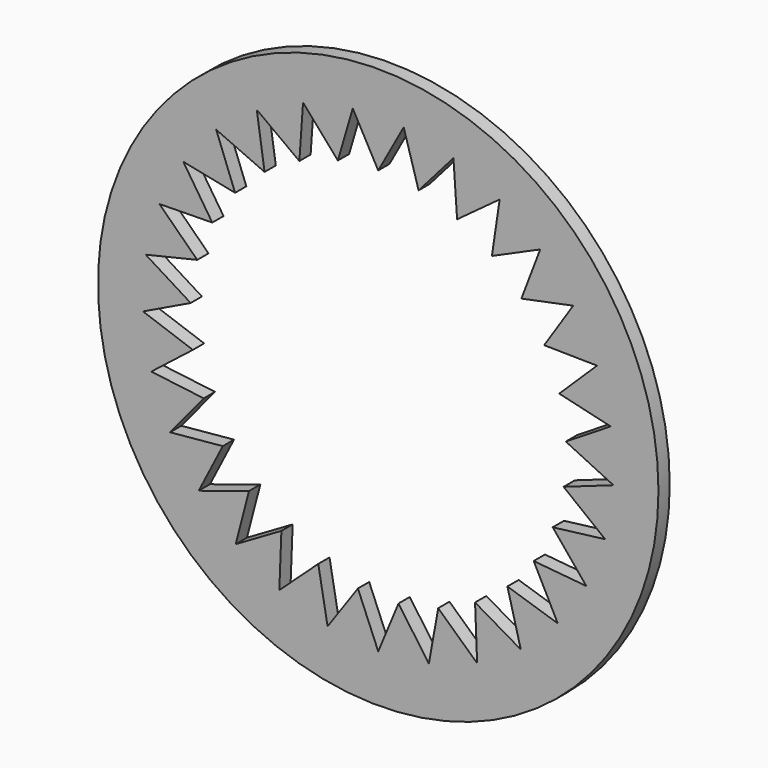
from build123d import *

# Parameters (mm, degrees)
F0_R     = 59.69
F1_DEPTH = 3


# Not quite as in the source:
# - a feature names something its author has since deleted; it is built from what else it names


with BuildPart() as f1:
    # F0 (on Front) → F1 (new body)
    with BuildSketch(Plane.XZ):
        Circle(F0_R)
        Polygon((-5.4242289373, 50.5095806797), (0, 40.6400127475), (5.4242289373, 50.5095806797), (8.5999770533, 39.7047088787), (16.0190558954, 48.1774829148), (16.7978287377, 36.9425310416), (25.8648496037, 43.6223336845), (24.2102326198, 32.482635602), (34.5012316912, 37.0571267042), (30.4905929324, 26.5335623138), (41.5243745303, 28.7888437555), (35.3452470073, 19.3734832321), (46.6058837673, 19.2041005596), (38.5471966155, 11.3371956968), (49.5081536781, 8.7510690557), (39.9467221522, 2.8004675814), (50.0954773473, -2.0814786208), (39.4783833586, -5.8375331953), (48.3403921728, -12.7870245801), (37.1640792362, -14.1729033174), (44.3249639868, -22.8649893915), (33.1120240736, -21.8158901421), (38.2369497485, -31.8441386213), (27.5116874668, -28.4091161002), (30.3610182372, -39.304617231), (20.624934931, -33.6442892735), (21.065439257, -44.8975815327), (12.7737833608, -37.2766187831), (10.7848637497, -48.3615107316), (4.3253438778, -39.136260938), (0, -49.5344353485), (-4.3253438778, -39.136260938), (-10.7848637497, -48.3615107316), (-12.7737833608, -37.2766187831), (-21.065439257, -44.8975815327), (-20.624934931, -33.6442892735), (-30.3610182372, -39.304617231), (-27.5116874668, -28.4091161002), (-38.2369497485, -31.8441386213), (-33.1120240736, -21.8158901421), (-44.3249639868, -22.8649893915), (-37.1640792362, -14.1729033174), (-48.3403921728, -12.7870245801), (-39.4783833586, -5.8375331953), (-50.0954773473, -2.0814786208), (-39.9467221522, 2.8004675814), (-49.5081536781, 8.7510690557), (-38.5471966155, 11.3371956968), (-46.6058837673, 19.2041005596), (-35.3452470073, 19.3734832321), (-41.5243745303, 28.7888437555), (-30.4905929324, 26.5335623138), (-34.5012316912, 37.0571267042), (-24.2102326198, 32.482635602), (-25.8648496037, 43.6223336845), (-16.7978287377, 36.9425310416), (-16.0190558954, 48.1774829148), (-8.5999770533, 39.7047088787), align=None, mode=Mode.SUBTRACT)
    extrude(amount=F1_DEPTH)


solid = f1.part
